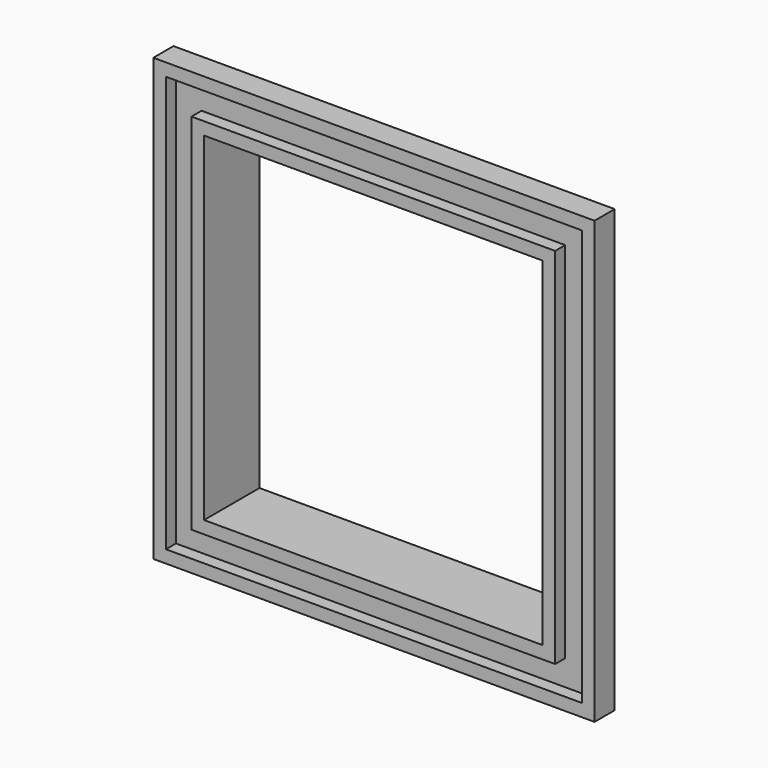
from build123d import *

# Parameters (mm, degrees)
F0_W        = 70
F0_H        = 70
F0_W_2      = 64.5
F0_H_2      = 64.5
F0_W_3      = 57.5
F0_H_3      = 57.5
F0_W_4      = 53.7
F0_H_4      = 53.7
F1_DEPTH    = 11
F2_DEPTH    = 7
F3_T        = 2
F3_T3_DEPTH = 61.5
F3_T5_DEPTH = 61.5
F3_T7_DEPTH = 15


# Not quite as in the source:
# - a shell that OpenCascade refuses in one call is made with other operations: the cavity is built on its own and cut out


with BuildPart() as f1:
    # F0 (on Front) → F1 (new body)
    with BuildSketch(Plane.XZ):
        with Locations((35, 35)):
            Rectangle(F0_W, F0_H)
        with Locations((35, 35)):
            Rectangle(F0_W_2, F0_H_2, mode=Mode.SUBTRACT)
        with Locations((35, 35)):
            Rectangle(F0_W_2, F0_H_2)
        with Locations((34.9, 34.9)):
            Rectangle(F0_W_3, F0_H_3, mode=Mode.SUBTRACT)
        with Locations((34.9, 34.9)):
            Rectangle(F0_W_3, F0_H_3)
        with Locations((34.9, 34.9)):
            Rectangle(F0_W_4, F0_H_4, mode=Mode.SUBTRACT)
    extrude(amount=F1_DEPTH)

    # F0 (on Front) → F2 (cut)
    with BuildSketch(Plane.XZ):
        with Locations((35, 35)):
            Rectangle(F0_W, F0_H)
        with Locations((35, 35)):
            Rectangle(F0_W_2, F0_H_2, mode=Mode.SUBTRACT)
        with Locations((35, 35)):
            Rectangle(F0_W_2, F0_H_2)
        with Locations((34.9, 34.9)):
            Rectangle(F0_W_3, F0_H_3, mode=Mode.SUBTRACT)
    extrude(amount=F2_DEPTH, mode=Mode.SUBTRACT)

    # F3: shell of thickness 2, made by hand


with BuildPart() as f3_core1:
    # F3_t2: copy of F1
    add(f1.part)

    # the walls: a layer under each face that stays
    f3_faces = [f3_core1.faces().sort_by_distance(p)[0] for p in [
        (0, -9, 35),
        (5, -7, 5),
        (35, -9, 0),
        (35, -9, 70),
        (70, -9, 35),
        (63.65, -3.5, 34.9),
        (34.9, -3.5, 6.15),
        (6.15, -3.5, 34.9),
        (34.9, -3.5, 63.65),
        (34.9, -5.5, 8.05),
        (8.05, -5.5, 34.9),
        (34.9, -5.5, 61.75),
        (61.75, -5.5, 34.9),
        (7.946875, 0, 40.2240740741),
    ]]
    thicken(f3_faces, amount=-F3_T, mode=Mode.SUBTRACT)

    # F3_s4 → F3_t3 (cut)
    with BuildSketch(Plane.XY.offset(4.15)):
        Polygon((63.67, -6.98), (63.65, -9), (61.65, -9), (61.65, -7), align=None)
        Polygon((6.13, -6.98), (6.15, -9), (8.15, -9), (8.15, -7), align=None)
    extrude(amount=F3_T3_DEPTH, mode=Mode.SUBTRACT)

    # F3_s6 → F3_t5 (cut)
    with BuildSketch(Plane.YZ.offset(4.15)):
        Polygon((-6.98, 6.13), (-9, 6.15), (-9, 8.15), (-7, 8.15), align=None)
        Polygon((-6.98, 63.67), (-9, 63.65), (-9, 61.65), (-7, 61.65), align=None)
    extrude(amount=F3_T5_DEPTH, mode=Mode.SUBTRACT)

    # F3_s8 → F3_t7 (cut)
    with BuildSketch(Plane.XZ.offset(-2)):
        Polygon((61.73, 8.07), (61.75, 6.05), (63.75, 6.05), (63.75, 8.05), align=None)
        Polygon((8.07, 8.07), (8.05, 6.05), (6.05, 6.05), (6.05, 8.05), align=None)
        Polygon((8.07, 61.73), (6.05, 61.75), (6.05, 63.75), (8.05, 63.75), align=None)
        Polygon((61.73, 61.73), (61.75, 63.75), (63.75, 63.75), (63.75, 61.75), align=None)
    extrude(amount=F3_T7_DEPTH, mode=Mode.SUBTRACT)


with BuildPart() as f1_1:
    add(f1.part)

    # what is left inside the walls is the cavity
    f3_cavity = [f3_core1.part.solids().sort_by_distance(p)[0] for p in [
        (39.125, -9.02, 4.444444),
    ]]
    add(f3_cavity, mode=Mode.SUBTRACT)


solid = f1_1.part
